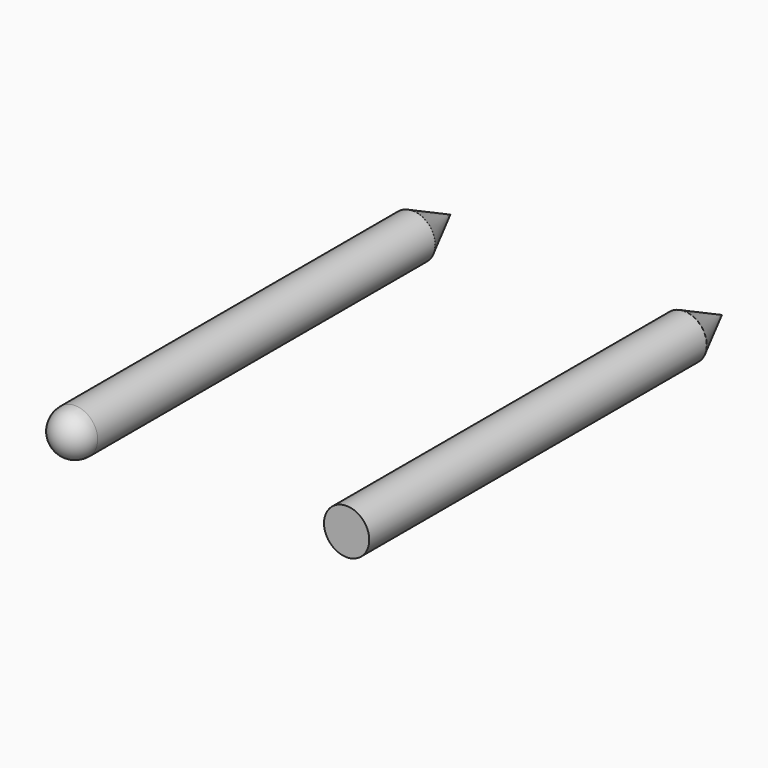
from build123d import *


# Not quite as in the source:
# - the program builds the solid bodies; features that only make, move or delete a surface that nothing else refers to are left out


with BuildPart() as f1:
    # F0 (on Top) → F1 (revolve)
    with BuildSketch(Plane.XY):
        Polygon((-23.5786662051, -47.3545584765), (-23.5786662051, 47.3545584765), (-28.6586662051, 57.9565837979), (-28.6586662051, 47.3545584765), (-28.6586662051, -47.3545584765), align=None)
    revolve(axis=Axis((-28.6586662051, 0, 0), (0, 1, 0)))

    # F0 (on Top) → F4 (revolve)
    with BuildSketch(Plane.XY):
        with BuildLine():
            ThreePointArc((-33.7386662051, -47.3545584765), (-28.6586662051, -52.4345584765), (-23.5786662051, -47.3545584765))
            Line((-23.5786662051, -47.3545584765), (-28.6586662051, -47.3545584765))
            Line((-28.6586662051, -47.3545584765), (-33.7386662051, -47.3545584765))
        make_face()
    revolve(axis=Axis((-28.6586662051, -47.3545584765, 0), (1, 0, 0)))


with BuildPart() as f2:
    # F0 (on Top) → F2 (revolve)
    with BuildSketch(Plane.XY):
        Polygon((32.3013337949, 57.9565837979), (27.2213337949, 47.3545584765), (27.2213337949, -47.3545584765), (32.3013337949, -47.3545584765), (32.3013337949, 47.3545584765), align=None)
    revolve(axis=Axis((32.3013337949, 0, 0), (0, -1, 0)))


solid = Compound([f1.part, f2.part])
